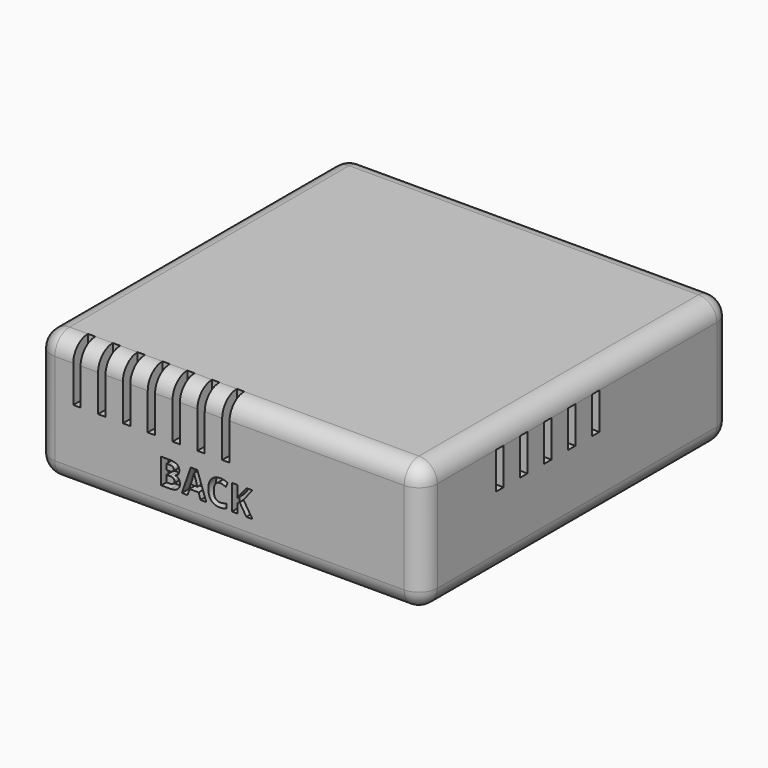
from build123d import *

# Parameters (mm, degrees)
F0_W         = 210
F0_H         = 210
F1_DEPTH     = 70
F2_R         = 10
F3_R         = 10
F4_W         = 4
F4_H         = 30
F5_DEPTH     = 10
F6_W         = 5
F6_H         = 20
F7_DEPTH     = 5
F8_TEXT_SIZE = 19.2795802529
F9_DEPTH     = 5
F10_R        = 10
F11_DEPTH    = 2


# Not quite as in the source:
# - a fillet or chamfer that OpenCascade refuses, or shapes differently, is made with other operations: its cross-section is extruded or revolved along the edge and cut away or added
# - Text() gives the source's letters only with a copy of the font that has no kerning and outlines rounded to 1/6400 em; it was checked with that copy


with BuildPart() as f1:
    # F0 (on Top) → F1 (new body)
    with BuildSketch(Plane.XY):
        Rectangle(F0_W, F0_H)
    extrude(amount=F1_DEPTH)

    # F2
    f2_edges = [f1.edges().sort_by_distance(p)[0] for p in [
        (-105, 105, 35),
        (105, 105, 35),
        (-105, -105, 35),
        (105, -105, 35),
    ]]
    fillet(f2_edges, radius=F2_R)

    # F3
    f3_edges = [f1.edges().sort_by_distance(p)[0] for p in [
        (105, 0, 70),
        (105, 0, 0),
        (102.071068, -102.071068, 0),
        (102.071068, 102.071068, 0),
        (0, -105, 0),
        (0, 105, 0),
        (-102.071068, -102.071068, 0),
        (-102.071068, 102.071068, 0),
        (-105, 0, 0),
        (102.071068, -102.071068, 70),
        (102.071068, 102.071068, 70),
        (0, 105, 70),
        (-102.071068, -102.071068, 70),
        (-102.071068, 102.071068, 70),
        (-105, 0, 70),
    ]]
    fillet(f3_edges, radius=F3_R)

    # F4 (on face) → F5 (cut)
    with BuildSketch(Plane.XZ.offset(105)):
        with Locations((-83, 55)):
            Rectangle(F4_W, F4_H)
        with Locations((-2, 55)):
            Rectangle(F4_W, F4_H)
        with Locations((-69.5, 55)):
            Rectangle(F4_W, F4_H)
        with Locations((-56, 55)):
            Rectangle(F4_W, F4_H)
        with Locations((-42.5, 55)):
            Rectangle(F4_W, F4_H)
        with Locations((-29, 55)):
            Rectangle(F4_W, F4_H)
        with Locations((-15.5, 55)):
            Rectangle(F4_W, F4_H)
    extrude(amount=-F5_DEPTH, mode=Mode.SUBTRACT)

    # F6 (on face) → F7 (cut)
    with BuildSketch(Plane.YZ.offset(105)):
        with Locations((-52.5, 50)):
            Rectangle(F6_W, F6_H)
        with Locations((-36.2, 50)):
            Rectangle(F6_W, F6_H)
        with Locations((-19.9, 50)):
            Rectangle(F6_W, F6_H)
        with Locations((-3.6, 50)):
            Rectangle(F6_W, F6_H)
        with Locations((12.7, 50)):
            Rectangle(F6_W, F6_H)
    extrude(amount=-F7_DEPTH, mode=Mode.SUBTRACT)

    # F8 (on face) → F9 (cut)
    with BuildSketch(Plane.XZ.offset(105)):
        with Locations((-38.9220751822, 17.0359667391)):
            Text('BACK', F8_TEXT_SIZE, font='Open Sans', font_style=FontStyle.BOLD, text_align=(TextAlign.LEFT, TextAlign.BOTTOM))
    extrude(amount=-F9_DEPTH, mode=Mode.SUBTRACT)

    # F10 (on face) → F11 (join)
    with BuildSketch(Plane(origin=(0, 105, 0), x_dir=(-1, 0, 0), z_dir=(0, 1, 0))):
        with Locations((-75, 40)):
            Circle(F10_R)
    extrude(amount=F11_DEPTH)

    # F12: fillet of radius 5 on 1 edges, made by hand

    # F12_s1 → F12_t2 (revolve, cut)
    with BuildSketch(Plane.XY.offset(40)):
        with BuildLine():
            ThreePointArc((65, 105), (66.7639320225, 106.472135955), (69, 107))
            Line((69, 107), (65, 107))
            Line((65, 107), (65, 105))
        make_face()
    revolve(axis=Axis((75, 107, 40), (0, 1, 0)), mode=Mode.SUBTRACT)


solid = f1.part
